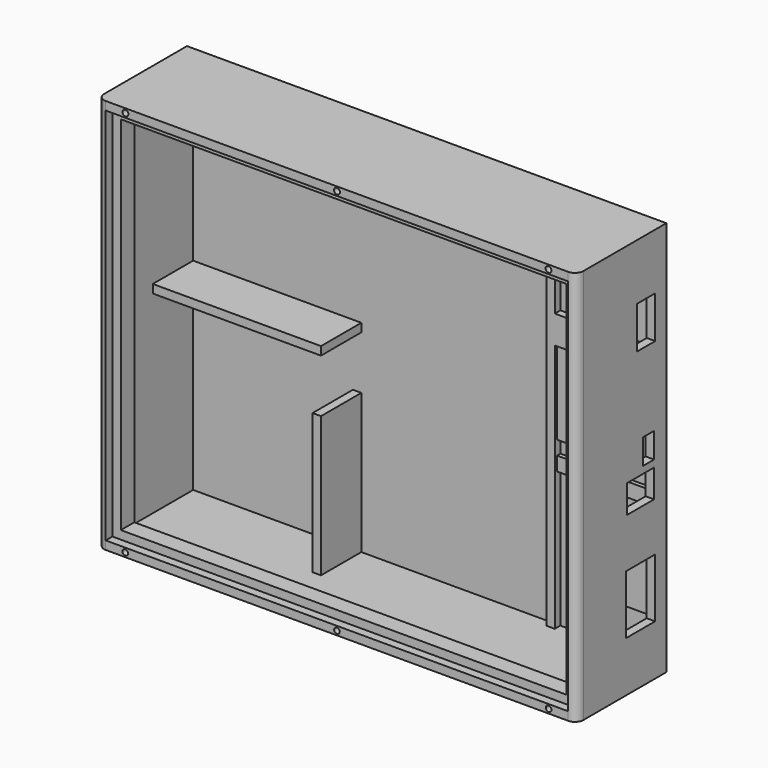
from build123d import *

# Parameters (mm, degrees)
F0_W      = 171
F0_H      = 141
F1_DEPTH  = 40
F2_W      = 82.5
F2_H      = 67.5
F3_DEPTH  = 3
F4_W      = 80.5
F4_H      = 65.5
F5_DEPTH  = 3
F6_W      = 82.5
F6_H      = 67.5
F7_DEPTH  = 36
F9_START  = 30
F9_DEPTH  = 6
F11_DEPTH = 39.9
F12_R     = 2.99999
F13_R     = 2.99999
F15_DEPTH = 87.6
F17_DEPTH = 58
F19_DEPTH = 2.5
F20_W     = 34
F20_H     = 30
F20_H_2   = 5
F21_DEPTH = 1.5
F22_W     = 22
F22_H     = 36
F23_DEPTH = 1
F25_DEPTH = 107.7
F27_DEPTH = 2
F29_DEPTH = 18
F31_DEPTH = 6
F33_DEPTH = 6


# Not quite as in the source:
# - a fillet or chamfer is up to 0.001 mm smaller than in the source, because OpenCascade refuses the exact size


with BuildPart() as f1:
    # F0 (on Front) → F1 (new body)
    with BuildSketch(Plane.XZ):
        with Locations((85.5, 70.5)):
            Rectangle(F0_W, F0_H)
    extrude(amount=F1_DEPTH)

    # F2 (on face) → F3 (cut)
    with BuildSketch(Plane.XZ.offset(40)):
        with Locations((126.75, 104.25)):
            Rectangle(F2_W, F2_H)
        with Locations((44.25, 104.25)):
            Rectangle(F2_W, F2_H)
        with Locations((126.75, 36.75)):
            Rectangle(F2_W, F2_H)
        with Locations((44.25, 36.75)):
            Rectangle(F2_W, F2_H)
    extrude(amount=-F3_DEPTH, mode=Mode.SUBTRACT)

    # F4 (on face) → F5 (cut)
    with BuildSketch(Plane.XZ.offset(37)):
        with Locations((45.25, 103.25)):
            Rectangle(F4_W, F4_H)
        with Locations((125.75, 103.25)):
            Rectangle(F4_W, F4_H)
        with Locations((125.75, 37.75)):
            Rectangle(F4_W, F4_H)
        with Locations((45.25, 37.75)):
            Rectangle(F4_W, F4_H)
    extrude(amount=-F5_DEPTH, mode=Mode.SUBTRACT)

    # F6 (on face) → F7 (cut)
    with BuildSketch(Plane.XZ.offset(37)):
        with Locations((126.75, 104.25)):
            Rectangle(F6_W, F6_H)
        with Locations((44.25, 104.25)):
            Rectangle(F6_W, F6_H)
        with Locations((126.75, 36.75)):
            Rectangle(F6_W, F6_H)
        with Locations((44.25, 36.75)):
            Rectangle(F6_W, F6_H)
    extrude(amount=-F7_DEPTH, mode=Mode.SUBTRACT)

    # F8 (on face) → F9 (join)
    with BuildSketch(Plane.XZ.offset(1).offset(F9_START)):
        Polygon((3, 138), (3, 70.5), (6, 70.5), (6, 135), (85.5, 135), (85.5, 138), align=None)
        Polygon((3, 70.5), (3, 3), (85.5, 3), (85.5, 6), (6, 6), (6, 70.5), align=None)
        Polygon((85.5, 6), (85.5, 3), (168, 3), (168, 70.5), (165, 70.5), (165, 6), align=None)
        Polygon((165, 70.5), (168, 70.5), (168, 138), (85.5, 138), (85.5, 135), (165, 135), align=None)
    extrude(amount=F9_DEPTH)

    # F10 (on face) → F11 (cut)
    with BuildSketch(Plane.YZ.offset(171)):
        Polygon((-13, 121), (-13, 106), (-5, 106), (-5, 113.5), (-5, 121), (-9, 121), align=None)
    extrude(amount=-F11_DEPTH, mode=Mode.SUBTRACT)

    # F12 (radius 3 in the source; OpenCascade refuses exactly that, so slightly less here)
    f12_edges = [f1.edges().sort_by_distance(p)[0] for p in [
        (171, -40, 70.5),
    ]]
    fillet(f12_edges, radius=F12_R)

    # F13 (radius 3 in the source; OpenCascade refuses exactly that, so slightly less here)
    f13_edges = [f1.edges().sort_by_distance(p)[0] for p in [
        (0, -40, 70.5),
    ]]
    fillet(f13_edges, radius=F13_R)

    # F14 (on face) → F15 (cut)
    with BuildSketch(Plane.YZ.offset(171)):
        Polygon((-10.5, 78), (-10.5, 69), (-5.5, 69), (-5.5, 73.5), (-5.5, 78), (-8, 78), align=None)
    extrude(amount=-F15_DEPTH, mode=Mode.SUBTRACT)

    # F16 (on face) → F17 (cut)
    with BuildSketch(Plane.YZ.offset(171)):
        Polygon((-17.5, 66.5), (-17.5, 56.5), (-5.5, 56.5), (-5.5, 61.5), (-5.5, 66.5), (-11.5, 66.5), align=None)
    extrude(amount=-F17_DEPTH, mode=Mode.SUBTRACT)

    # F18 (on face) → F19 (join)
    with BuildSketch(Plane.XZ.offset(1)):
        Polygon((134, 138), (131, 138), (131, 3), (134, 3), (134, 70.5), (134, 92), (134, 102), align=None)
        Polygon((151, 102), (134, 102), (134, 92), (168, 92), (168, 102), align=None)
    extrude(amount=F19_DEPTH)

    # F20 (on face) → F21 (join)
    with BuildSketch(Plane.XZ.offset(1)):
        with Locations((151, 77)):
            Rectangle(F20_W, F20_H)
        with Locations((151, 54.5)):
            Rectangle(F20_W, F20_H_2)
    extrude(amount=F21_DEPTH)

    # F22 (on face) → F23 (join)
    with BuildSketch(Plane.XZ.offset(1)):
        with Locations((157, 120)):
            Rectangle(F22_W, F22_H)
    extrude(amount=F23_DEPTH)

    # F24 (on face) → F25 (cut)
    with BuildSketch(Plane.YZ.offset(171)):
        Polygon((-18, 39), (-18, 18), (-11.5, 18), (-5, 18), (-5, 28.5), (-5, 39), align=None)
    extrude(amount=-F25_DEPTH, mode=Mode.SUBTRACT)

    # F26 (on face) → F27 (join)
    with BuildSketch(Plane.XZ.offset(1)):
        Polygon((168, 18), (168, 38), (153, 38), (153, 18), (160.5, 18), align=None)
    extrude(amount=F27_DEPTH)

    # F28 (on face) → F29 (join)
    with BuildSketch(Plane.XZ.offset(1)):
        Polygon((60, 53), (60, 28), (60, 3), (63, 3), (63, 53), align=None)
        Polygon((63, 75), (3, 75), (3, 72), (33, 72), (63, 72), align=None)
    extrude(amount=F29_DEPTH)

    # F30 (on face) → F31 (cut)
    with BuildSketch(Plane.XZ.offset(40)):
        with BuildLine():
            Line((10.05, 139.5), (9, 139.5))
            ThreePointArc((9, 139.5), (10.05, 138.45), (11.1, 139.5))
            Line((11.1, 139.5), (10.05, 139.5))
        make_face()
        with BuildLine():
            ThreePointArc((160.95, 140.55), (160.2075378798, 140.2424621202), (159.9, 139.5))
            Line((159.9, 139.5), (160.95, 139.5))
            Line((160.95, 139.5), (160.95, 140.55))
        make_face()
        with BuildLine():
            Line((160.95, 139.5), (159.9, 139.5))
            ThreePointArc((159.9, 139.5), (160.95, 138.45), (162, 139.5))
            Line((162, 139.5), (160.95, 139.5))
        make_face()
        with BuildLine():
            ThreePointArc((86.55, 139.5), (85.5, 140.55), (84.45, 139.5))
            Line((84.45, 139.5), (86.55, 139.5))
        make_face()
        with BuildLine():
            Line((86.55, 139.5), (84.45, 139.5))
            ThreePointArc((84.45, 139.5), (85.5, 138.45), (86.55, 139.5))
        make_face()
        with BuildLine():
            ThreePointArc((10.05, 140.55), (9.3075378798, 140.2424621202), (9, 139.5))
            Line((9, 139.5), (10.05, 139.5))
            Line((10.05, 139.5), (10.05, 140.55))
        make_face()
        with BuildLine():
            Line((10.05, 139.5), (11.1, 139.5))
            ThreePointArc((11.1, 139.5), (10.7924621202, 140.2424621202), (10.05, 140.55))
            Line((10.05, 140.55), (10.05, 139.5))
        make_face()
        with BuildLine():
            ThreePointArc((162, 139.5), (161.6924621202, 140.2424621202), (160.95, 140.55))
            Line((160.95, 140.55), (160.95, 139.5))
            Line((160.95, 139.5), (162, 139.5))
        make_face()
    extrude(amount=-F31_DEPTH, mode=Mode.SUBTRACT)

    # F32 (on face) → F33 (cut)
    with BuildSketch(Plane.XZ.offset(40)):
        with BuildLine():
            Line((10, 1.5), (9, 1.5))
            ThreePointArc((9, 1.5), (10, 0.5), (11, 1.5))
            Line((11, 1.5), (10, 1.5))
        make_face()
        with BuildLine():
            ThreePointArc((161, 2.5), (160.2928932188, 2.2071067812), (160, 1.5))
            Line((160, 1.5), (161, 1.5))
            Line((161, 1.5), (161, 2.5))
        make_face()
        with BuildLine():
            Line((161, 1.5), (160, 1.5))
            ThreePointArc((160, 1.5), (161, 0.5), (162, 1.5))
            Line((162, 1.5), (161, 1.5))
        make_face()
        with BuildLine():
            ThreePointArc((86.5, 1.5), (85.5, 2.5), (84.5, 1.5))
            Line((84.5, 1.5), (86.5, 1.5))
        make_face()
        with BuildLine():
            Line((86.5, 1.5), (84.5, 1.5))
            ThreePointArc((84.5, 1.5), (85.5, 0.5), (86.5, 1.5))
        make_face()
        with BuildLine():
            ThreePointArc((10, 2.5), (9.2928932188, 2.2071067812), (9, 1.5))
            Line((9, 1.5), (10, 1.5))
            Line((10, 1.5), (10, 2.5))
        make_face()
        with BuildLine():
            Line((10, 1.5), (11, 1.5))
            ThreePointArc((11, 1.5), (10.7071067812, 2.2071067812), (10, 2.5))
            Line((10, 2.5), (10, 1.5))
        make_face()
        with BuildLine():
            ThreePointArc((162, 1.5), (161.7071067812, 2.2071067812), (161, 2.5))
            Line((161, 2.5), (161, 1.5))
            Line((161, 1.5), (162, 1.5))
        make_face()
    extrude(amount=-F33_DEPTH, mode=Mode.SUBTRACT)


solid = f1.part
